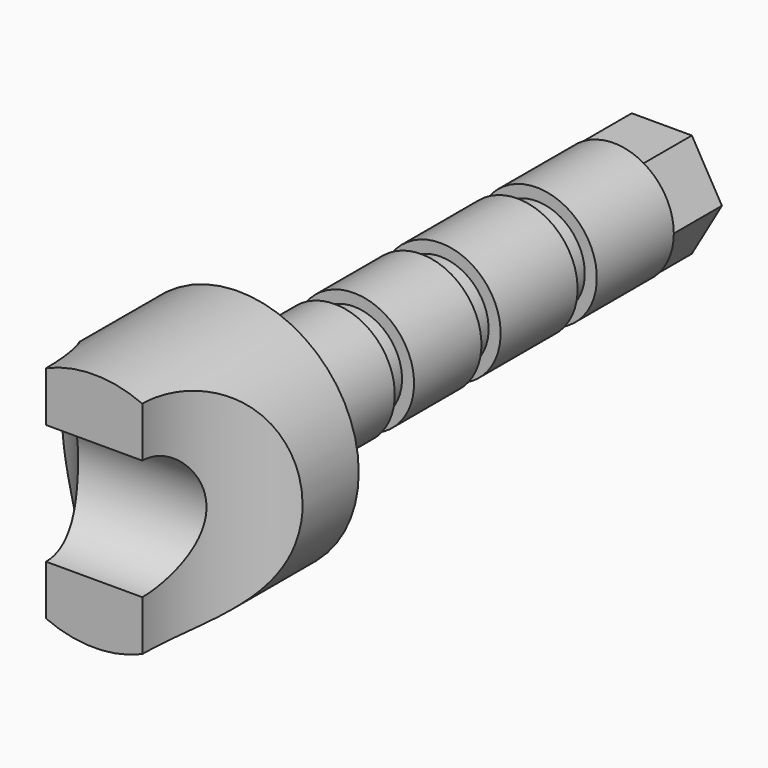
from build123d import *

# Parameters (mm, degrees)
F0_R      = 50
F1_DEPTH  = 75
F2_R      = 25
F3_DEPTH  = 50
F4_R      = 20
F5_DEPTH  = 10
F6_R      = 25
F7_DEPTH  = 35
F8_R      = 20
F9_DEPTH  = 10
F10_R     = 25
F11_DEPTH = 40
F12_R     = 20
F13_DEPTH = 10
F14_R     = 25
F15_DEPTH = 40
F17_DEPTH = 25
F19_ANGLE = 90
F22_R     = 25
F23_DEPTH = 50


# Not quite as in the source:
# - a feature names something its author has since deleted; it is built from what else it names


with BuildPart() as f1:
    # F0 (on Front) → F1 (new body)
    with BuildSketch(Plane.XZ):
        Circle(F0_R)
    extrude(amount=F1_DEPTH)

    # F2 (on face) → F3 (join)
    with BuildSketch(Plane(origin=(0, 0, 0), x_dir=(-1, 0, 0), z_dir=(0, 1, 0))):
        Circle(F2_R)
    extrude(amount=F3_DEPTH)

    # F4 (on face) → F5 (join)
    with BuildSketch(Plane(origin=(0, 50, 0), x_dir=(-1, 0, 0), z_dir=(0, 1, 0))):
        Circle(F4_R)
    extrude(amount=F5_DEPTH)

    # F6 (on face) → F7 (join)
    with BuildSketch(Plane(origin=(0, 60, 0), x_dir=(-1, 0, 0), z_dir=(0, 1, 0))):
        Circle(F6_R)
    extrude(amount=F7_DEPTH)

    # F8 (on face) → F9 (join)
    with BuildSketch(Plane(origin=(0, 95, 0), x_dir=(-1, 0, 0), z_dir=(0, 1, 0))):
        Circle(F8_R)
    extrude(amount=F9_DEPTH)

    # F10 (on face) → F11 (join)
    with BuildSketch(Plane(origin=(0, 105, 0), x_dir=(-1, 0, 0), z_dir=(0, 1, 0))):
        Circle(F10_R)
    extrude(amount=F11_DEPTH)

    # F12 (on face) → F13 (join)
    with BuildSketch(Plane(origin=(0, 145, 0), x_dir=(-1, 0, 0), z_dir=(0, 1, 0))):
        Circle(F12_R)
    extrude(amount=F13_DEPTH)

    # F14 (on face) → F15 (join)
    with BuildSketch(Plane(origin=(0, 155, 0), x_dir=(-1, 0, 0), z_dir=(0, 1, 0))):
        Circle(F14_R)
    extrude(amount=F15_DEPTH)

    # F16 (on face) → F17 (join)
    with BuildSketch(Plane(origin=(0, 195, 0), x_dir=(-1, 0, 0), z_dir=(0, 1, 0))):
        Polygon((12.5, 21.6506350946), (-12.5, 21.6506350946), (-25, 0), (-12.5, -21.6506350946), (12.5, -21.6506350946), (25, 0), align=None)
    extrude(amount=F17_DEPTH)

    # F18 (on face) → F19 (revolve, cut)
    with BuildSketch(Plane.XZ.offset(75)):
        with BuildLine():
            ThreePointArc((50, 0), (41.8330013267, 27.3861278753), (20, 45.8257569496))
            Line((20, 45.8257569496), (20, -45.8257569496))
            ThreePointArc((20, -45.8257569496), (41.8330013267, -27.3861278753), (50, 0))
        make_face()
    revolve(axis=Axis((70, -75, -0.5619522762), (0, 0, -1)), revolution_arc=F19_ANGLE, mode=Mode.SUBTRACT)

    # F20 (on face) → F21 (revolve, cut)
    with BuildSketch(Plane.XZ.offset(75)):
        with BuildLine():
            Line((-20, -45.8257569496), (-20, 45.8257569496))
            ThreePointArc((-20, 45.8257569496), (-50, 0), (-20, -45.8257569496))
        make_face()
    revolve(axis=Axis((-70, -75, -0.6762938916), (0, 0, -1)), mode=Mode.SUBTRACT)

    # F22 (on Right) → F23 (cut, symmetric)
    with BuildSketch(Plane.YZ):
        with Locations((-75, 0)):
            Circle(F22_R)
    extrude(amount=F23_DEPTH, both=True, mode=Mode.SUBTRACT)


solid = f1.part
